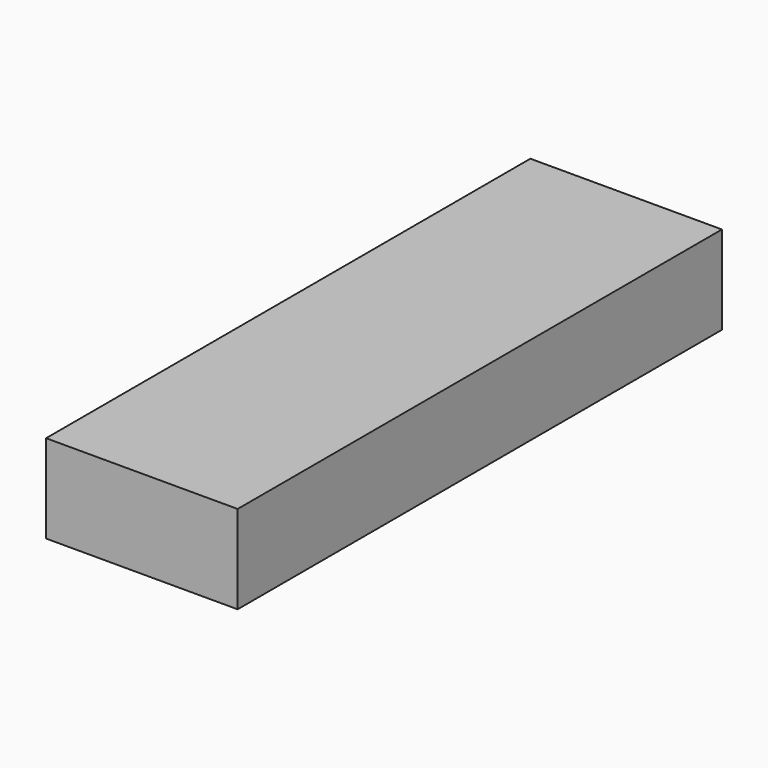
from build123d import *

# Parameters (mm, degrees)
F1_W     = 55.0690628588
F1_H     = 174.0121990442
F2_DEPTH = 25.4


# Not quite as in the source:
# - the program builds the solid bodies; features that only make, move or delete a surface that nothing else refers to are left out


with BuildPart() as f2:
    # F1 (on Top) → F2 (new body)
    with BuildSketch(Plane.XY):
        with Locations((-27.5345314294, 87.0060995221)):
            Rectangle(F1_W, F1_H)
    extrude(amount=F2_DEPTH)


solid = f2.part
